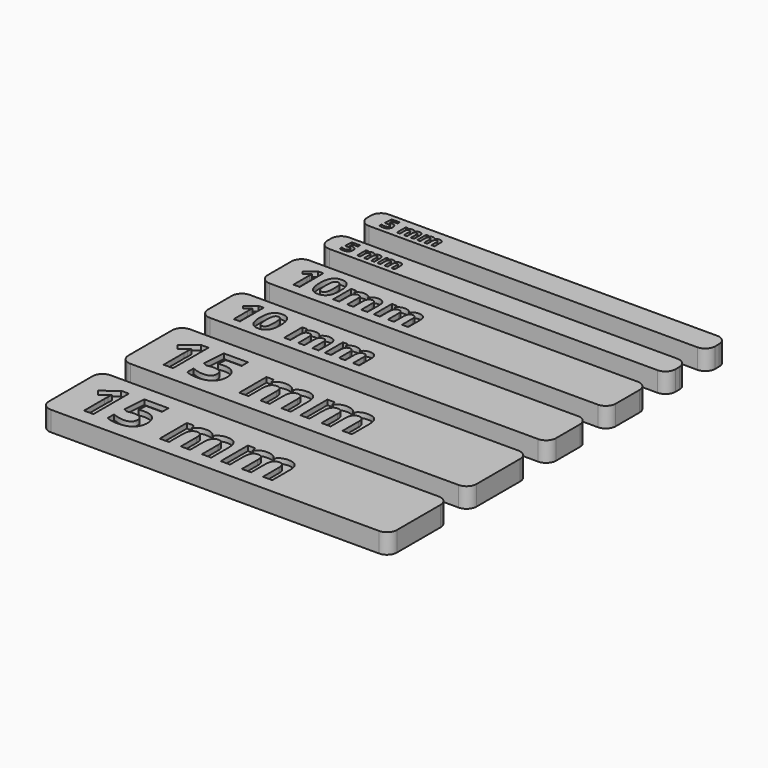
from build123d import *

# Parameters (mm, degrees)
F0_W           = 70
F0_H           = 5
F1_DEPTH       = 4
F0_H_2         = 10
F0_H_3         = 15
F2_TEXT_SIZE   = 12.5
F2_TEXT_SIZE_2 = 8.3333333333
F2_TEXT_SIZE_3 = 4.1666666667
F3_DEPTH       = 1
F4_R           = 2
F4_2_R         = 2
F4_3_R         = 2
F4_4_R         = 2
F4_5_R         = 2
F4_6_R         = 2


# Not quite as in the source:
# - Text() gives the source's letters only with a copy of the font that has no kerning and outlines rounded to 1/6400 em; it was checked with that copy


with BuildPart() as f1:
    # F0 (on Top) → F1 (new body)
    with BuildSketch(Plane.XY):
        with Locations((0, 12.5)):
            Rectangle(F0_W, F0_H)
    extrude(amount=F1_DEPTH)


with BuildPart() as f1b:
    # F0 (on Top) → F1, piece 2 (new body)
    with BuildSketch(Plane.XY):
        with Locations((0, 2.5)):
            Rectangle(F0_W, F0_H)
    extrude(amount=F1_DEPTH)


with BuildPart() as f1c:
    # F0 (on Top) → F1, piece 3 (new body)
    with BuildSketch(Plane.XY):
        with Locations((0, -10)):
            Rectangle(F0_W, F0_H_2)
    extrude(amount=F1_DEPTH)


with BuildPart() as f1d:
    # F0 (on Top) → F1, piece 4 (new body)
    with BuildSketch(Plane.XY):
        with Locations((0, -25)):
            Rectangle(F0_W, F0_H_2)
    extrude(amount=F1_DEPTH)


with BuildPart() as f1e:
    # F0 (on Top) → F1, piece 5 (new body)
    with BuildSketch(Plane.XY):
        with Locations((0, -42.5)):
            Rectangle(F0_W, F0_H_3)
    extrude(amount=F1_DEPTH)


with BuildPart() as f1f:
    # F0 (on Top) → F1, piece 6 (new body)
    with BuildSketch(Plane.XY):
        with Locations((0, -62.5)):
            Rectangle(F0_W, F0_H_3)
    extrude(amount=F1_DEPTH)


with BuildPart() as f3_tool:
    # F2 (on face) → F3 (new body)
    with BuildSketch(Plane.XY.offset(4)):
        with Locations((-32, -67)):
            Text('15 mm', F2_TEXT_SIZE, font='Open Sans', font_style=FontStyle.BOLD, text_align=(TextAlign.LEFT, TextAlign.BOTTOM))
        with Locations((-32, -28)):
            Text('10 mm', F2_TEXT_SIZE_2, font='Open Sans', font_style=FontStyle.BOLD, text_align=(TextAlign.LEFT, TextAlign.BOTTOM))
        with Locations((-32, 1)):
            Text('5 mm', F2_TEXT_SIZE_3, font='Open Sans', font_style=FontStyle.BOLD, text_align=(TextAlign.LEFT, TextAlign.BOTTOM))
        with Locations((-32, -47)):
            Text('15 mm', F2_TEXT_SIZE, font='Open Sans', font_style=FontStyle.BOLD, text_align=(TextAlign.LEFT, TextAlign.BOTTOM))
        with Locations((-32, -13)):
            Text('10mm', F2_TEXT_SIZE_2, font='Open Sans', font_style=FontStyle.BOLD, text_align=(TextAlign.LEFT, TextAlign.BOTTOM))
        with Locations((-32, 11)):
            Text('5 mm', F2_TEXT_SIZE_3, font='Open Sans', font_style=FontStyle.BOLD, text_align=(TextAlign.LEFT, TextAlign.BOTTOM))
    extrude(amount=-F3_DEPTH)


with BuildPart() as f1_1:
    add(f1.part)

    # F3: cut by f3_tool
    add(f3_tool.part, mode=Mode.SUBTRACT)

    # F4
    f4_edges = [f1_1.edges().sort_by_distance(p)[0] for p in [
        (-35, 15, 2),
        (-35, 10, 2),
        (35, 15, 2),
        (35, 10, 2),
    ]]
    fillet(f4_edges, radius=F4_R)


with BuildPart() as f1b_1:
    add(f1b.part)

    # F3: cut by f3_tool
    add(f3_tool.part, mode=Mode.SUBTRACT)

    # F4#2
    f4_2_edges = [f1b_1.edges().sort_by_distance(p)[0] for p in [
        (-35, 5, 2),
        (-35, 0, 2),
        (35, 5, 2),
        (35, 0, 2),
    ]]
    fillet(f4_2_edges, radius=F4_2_R)


with BuildPart() as f1c_1:
    add(f1c.part)

    # F3: cut by f3_tool
    add(f3_tool.part, mode=Mode.SUBTRACT)

    # F4#3
    f4_3_edges = [f1c_1.edges().sort_by_distance(p)[0] for p in [
        (-35, -5, 2),
        (-35, -15, 2),
        (35, -5, 2),
        (35, -15, 2),
    ]]
    fillet(f4_3_edges, radius=F4_3_R)


with BuildPart() as f1d_1:
    add(f1d.part)

    # F3: cut by f3_tool
    add(f3_tool.part, mode=Mode.SUBTRACT)

    # F4#4
    f4_4_edges = [f1d_1.edges().sort_by_distance(p)[0] for p in [
        (-35, -20, 2),
        (-35, -30, 2),
        (35, -20, 2),
        (35, -30, 2),
    ]]
    fillet(f4_4_edges, radius=F4_4_R)


with BuildPart() as f1e_1:
    add(f1e.part)

    # F3: cut by f3_tool
    add(f3_tool.part, mode=Mode.SUBTRACT)

    # F4#5
    f4_5_edges = [f1e_1.edges().sort_by_distance(p)[0] for p in [
        (-35, -35, 2),
        (-35, -50, 2),
        (35, -35, 2),
        (35, -50, 2),
    ]]
    fillet(f4_5_edges, radius=F4_5_R)


with BuildPart() as f1f_1:
    add(f1f.part)

    # F3: cut by f3_tool
    add(f3_tool.part, mode=Mode.SUBTRACT)

    # F4#6
    f4_6_edges = [f1f_1.edges().sort_by_distance(p)[0] for p in [
        (-35, -55, 2),
        (-35, -70, 2),
        (35, -55, 2),
        (35, -70, 2),
    ]]
    fillet(f4_6_edges, radius=F4_6_R)


solid = Compound([f1_1.part, f1b_1.part, f1c_1.part, f1d_1.part, f1e_1.part, f1f_1.part])
